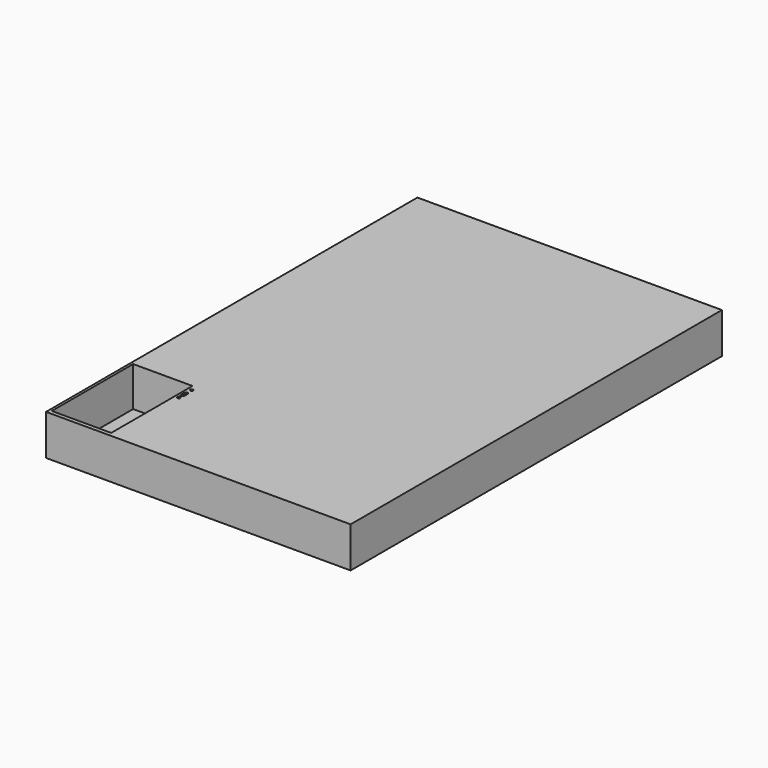
from build123d import *

# Parameters (mm, degrees)
F0_W     = 399.9802543244
F0_H     = 609.6
F1_DEPTH = 53.34
F2_W     = 78.0126031023
F2_H     = 133.5061052814
F3_DEPTH = 52.07
F4_W     = 133.5061052814
F4_H     = 51.0229802537
F5_DEPTH = 10.16
F6_R     = 1.8396087238
F6_R_2   = 1.9116150916
F7_DEPTH = 25.4


with BuildPart() as f1:
    # F0 (on Top) → F1 (new body)
    with BuildSketch(Plane.XY):
        with Locations((199.9901271622, 304.8)):
            Rectangle(F0_W, F0_H)
    extrude(amount=F1_DEPTH)

    # F2 (on face) → F3 (cut)
    with BuildSketch(Plane.XY.offset(53.34)):
        with Locations((42.3716591904, 71.9645838253)):
            Rectangle(F2_W, F2_H)
    extrude(amount=-F3_DEPTH, mode=Mode.SUBTRACT)

    # F4 (on face) → F5 (cut)
    with BuildSketch(Plane(origin=(81.3779607415, 0, 0), x_dir=(0, -1, 0), z_dir=(-1, 0, 0))):
        with Locations((-71.9645838253, 26.7814901268)):
            Rectangle(F4_W, F4_H)
    extrude(amount=-F5_DEPTH, mode=Mode.SUBTRACT)

    # F6 (on face) → F7 (cut)
    with BuildSketch(Plane.XY.offset(53.34)):
        with Locations((86.4754936327, 130.9549957514)):
            Circle(F6_R)
        with BuildLine():
            Line((84.4225700873, 121.4809922279), (84.4225700873, 117.0233345083))
            ThreePointArc((84.4225700873, 117.0233345083), (86.1374283625, 114.22337587), (88.6342981207, 116.3555458188))
            Line((88.6342981207, 116.3555458188), (88.6336831498, 116.4070708193))
            Line((88.6336831498, 116.4070708193), (88.5679829552, 121.9117257152))
            ThreePointArc((88.5679829552, 121.9117257152), (86.6669107252, 123.970616392), (84.4225700873, 122.2925098566))
            Line((84.4225700873, 122.2925098566), (84.4225700873, 121.4809922279))
        make_face()
        with Locations((86.4754936327, 110.0129559636)):
            Circle(F6_R_2)
    extrude(amount=-F7_DEPTH, mode=Mode.SUBTRACT)


solid = f1.part
